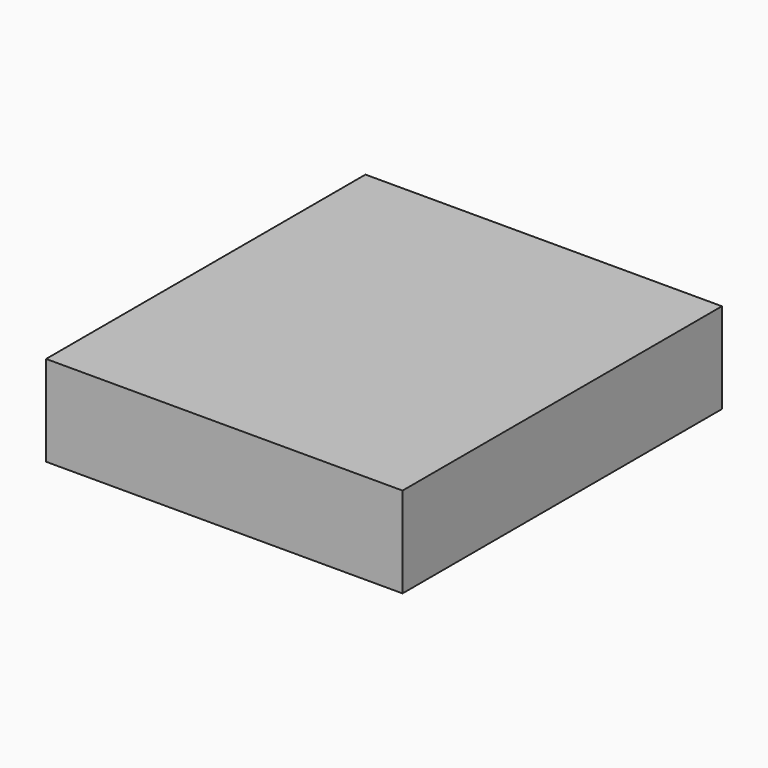
from build123d import *

# Parameters (mm, degrees)
F0_W     = 25
F0_H     = 28
F1_DEPTH = 6.35


# Not quite as in the source:
# - a length typed as a fraction of an inch, garbled in the dataset ("3 / 203.2 mm" for 3/8 in), is restored


with BuildPart() as f1:
    # F0 (on Top) → F1 (new body)
    with BuildSketch(Plane.XY):
        with Locations((-0.3986696121, 1.2061810121)):
            Rectangle(F0_W, F0_H)
    extrude(amount=F1_DEPTH)


solid = f1.part
